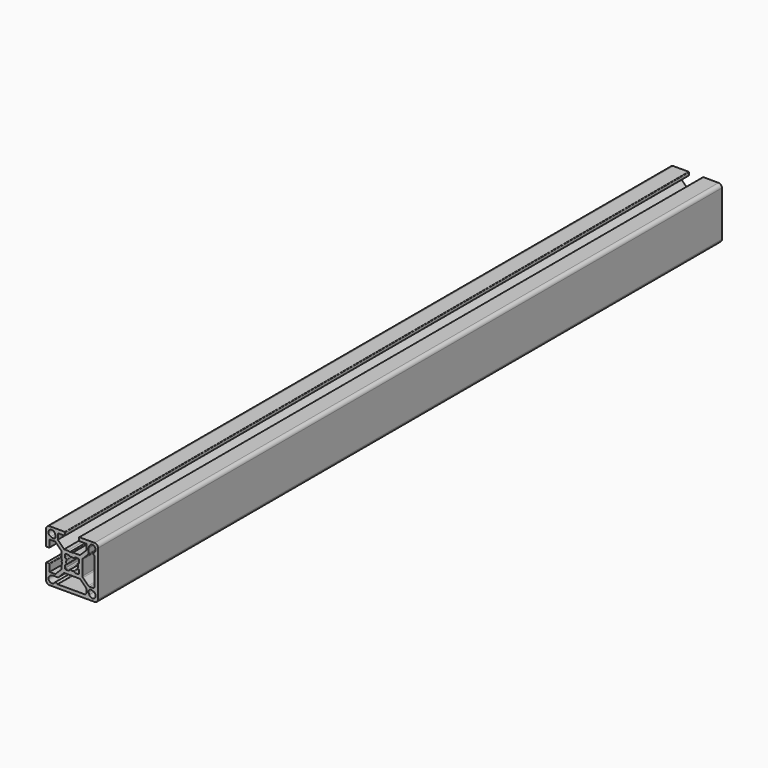
from build123d import *

# Parameters (mm, degrees)
F2_DEPTH = 225


# Not quite as in the source:
# - ends of sketch curves that miss each other by under 0.0002 mm in the source are joined


with BuildPart() as f2:
    # F1 (on Front) → F2 (new body, symmetric)
    with BuildSketch(Plane.XZ):
        with BuildLine():
            Line((-48.090856, 20.246586), (-44.140856, 20.246586))
            ThreePointArc((-44.140856, 20.246586), (-43.9287239656, 20.3344539656), (-43.840856, 20.546586))
            Line((-43.840856, 20.546586), (-43.840856, 21.946586))
            ThreePointArc((-43.840856, 21.946586), (-43.9287239656, 22.1587180344), (-44.140856, 22.246586))
            Line((-44.140856, 22.246586), (-52.840856, 22.246586))
            ThreePointArc((-52.840856, 22.246586), (-54.2550695624, 21.6607995624), (-54.840856, 20.246586))
            Line((-54.840856, 20.246586), (-54.840856, 11.546586))
            ThreePointArc((-54.840856, 11.546586), (-54.7529880344, 11.3344539656), (-54.540856, 11.246586))
            Line((-54.540856, 11.246586), (-53.140856, 11.246586))
            ThreePointArc((-53.140856, 11.246586), (-52.9287239656, 11.3344539656), (-52.840856, 11.546586))
            Line((-52.840856, 11.546586), (-52.840856, 15.496586))
            Line((-52.840856, 15.496586), (-49.50507, 15.496586))
            Line((-49.50507, 15.496586), (-45.840856, 11.832372))
            Line((-45.840856, 11.832372), (-45.840856, 7.900176))
            ThreePointArc((-45.840856, 7.900176), (-45.8238189324, 7.7707665494), (-45.7738687764, 7.6501761291))
            Line((-45.7738687764, 7.6501761291), (-45.540856, 7.246586))
            Line((-45.540856, 7.246586), (-45.773869, 6.842996))
            ThreePointArc((-45.773869, 6.842996), (-45.840856, 6.592996), (-45.7738687764, 6.3429961291))
            Line((-45.7738687764, 6.3429961291), (-45.591833, 6.0277))
            Line((-45.591833, 6.0277), (-45.840856, 4.746586))
            Line((-45.840856, 4.746586), (-45.840856, 2.6608))
            Line((-45.840856, 2.6608), (-49.50507, -1.003414))
            Line((-49.50507, -1.003414), (-52.840856, -1.003414))
            Line((-52.840856, -1.003414), (-52.840856, 2.946586))
            ThreePointArc((-52.840856, 2.946586), (-52.9287239656, 3.1587180344), (-53.140856, 3.246586))
            Line((-53.140856, 3.246586), (-54.540856, 3.246586))
            ThreePointArc((-54.540856, 3.246586), (-54.7529880344, 3.1587180344), (-54.840856, 2.946586))
            Line((-54.840856, 2.946586), (-54.840856, -5.753414))
            ThreePointArc((-54.840856, -5.753414), (-54.2550695624, -7.1676275624), (-52.840856, -7.753414))
            Line((-52.840856, -7.753414), (-26.840856, -7.753414))
            ThreePointArc((-26.840856, -7.753414), (-25.4266424376, -7.1676275624), (-24.840856, -5.753414))
            Line((-24.840856, -5.753414), (-24.840856, 20.246586))
            ThreePointArc((-24.840856, 20.246586), (-25.4266424376, 21.6607995624), (-26.840856, 22.246586))
            Line((-26.840856, 22.246586), (-35.540856, 22.246586))
            ThreePointArc((-35.540856, 22.246586), (-35.7529880344, 22.1587180344), (-35.840856, 21.946586))
            Line((-35.840856, 21.946586), (-35.840856, 20.546586))
            ThreePointArc((-35.840856, 20.546586), (-35.7529880344, 20.3344539656), (-35.540856, 20.246586))
            Line((-35.540856, 20.246586), (-31.590856, 20.246586))
            Line((-31.590856, 20.246586), (-31.590856, 16.9108))
            Line((-31.590856, 16.9108), (-35.25507, 13.246586))
            Line((-35.25507, 13.246586), (-39.187266, 13.246586))
            ThreePointArc((-39.187266, 13.246586), (-39.3166754506, 13.2295489324), (-39.4372658709, 13.1795987764))
            Line((-39.4372658709, 13.1795987764), (-39.840856, 12.946586))
            Line((-39.840856, 12.946586), (-40.244446, 13.179599))
            ThreePointArc((-40.244446, 13.179599), (-40.494446, 13.246586), (-40.7444458709, 13.1795987764))
            Line((-40.7444458709, 13.1795987764), (-41.059742, 12.997563))
            Line((-41.059742, 12.997563), (-42.340856, 13.246586))
            Line((-42.340856, 13.246586), (-44.426642, 13.246586))
            Line((-44.426642, 13.246586), (-48.090856, 16.9108))
            Line((-48.090856, 16.9108), (-48.090856, 20.246586))
        make_face()
        with BuildLine():
            ThreePointArc((-48.030175, -5.753414), (-48.180175082, -5.7132215738), (-48.2899827159, -5.6034138359))
            ThreePointArc((-48.2899827159, -5.6034138359), (-49.1151948384, -5.1042472042), (-49.9783690315, -5.5344479782))
            ThreePointArc((-49.9783690315, -5.5344479782), (-53.0449723505, -5.6142903949), (-52.1906940253, -2.6679979306))
            Line((-52.1906940253, -2.6679979306), (-50.91426, -2.203414))
            Line((-50.91426, -2.203414), (-48.290856, -2.203414))
            ThreePointArc((-48.290856, -2.203414), (-47.9081725676, -2.1272935325), (-47.5837492188, -1.9105207812))
            Line((-47.5837492188, -1.9105207812), (-44.719536, 0.953693))
            ThreePointArc((-44.719536, 0.953693), (-44.3951124324, 1.1704655325), (-44.012429, 1.246586))
            Line((-44.012429, 1.246586), (-35.669283, 1.246586))
            ThreePointArc((-35.669283, 1.246586), (-35.2865995676, 1.1704655325), (-34.9621762188, 0.9536927812))
            Line((-34.9621762188, 0.9536927812), (-31.883749, -2.124734))
            ThreePointArc((-31.883749, -2.124734), (-31.6669764675, -2.4491575676), (-31.590856, -2.831841))
            Line((-31.590856, -2.831841), (-31.590856, -4.753414))
            ThreePointArc((-31.590856, -4.753414), (-31.8837492188, -5.4605207812), (-32.590856, -5.753414))
            Line((-32.590856, -5.753414), (-48.030175, -5.753414))
        make_face(mode=Mode.SUBTRACT)
        with BuildLine():
            ThreePointArc((-30.2930043339, -4.0956641215), (-29.9673844937, -2.6268855063), (-28.4986058785, -2.3012656661))
            Line((-28.4986058785, -2.3012656661), (-27.491018, -2.667998))
            ThreePointArc((-27.491018, -2.667998), (-26.7973531157, -5.7969168843), (-29.9262720694, -5.1032520253))
            Line((-29.9262720694, -5.1032520253), (-30.2930043339, -4.0956641215))
        make_face(mode=Mode.SUBTRACT)
        with BuildLine():
            ThreePointArc((-36.5876690145, 8.2349049956), (-36.440856, 7.246586), (-36.5876690145, 6.2582670044))
            ThreePointArc((-36.5876690145, 6.2582670044), (-36.5433888407, 5.9288023569), (-36.2653470651, 5.7465855742))
            ThreePointArc((-36.2653470651, 5.7465855742), (-35.9615444769, 5.5780848975), (-35.840856, 5.25232))
            Line((-35.840856, 5.25232), (-35.840856, 3.746586))
            ThreePointArc((-35.840856, 3.746586), (-35.9873026094, 3.3930326094), (-36.340856, 3.246586))
            Line((-36.340856, 3.246586), (-37.84659, 3.246586))
            ThreePointArc((-37.84659, 3.246586), (-38.1723548975, 3.3672744769), (-38.3408555178, 3.6710770737))
            ThreePointArc((-38.3408555178, 3.6710770737), (-38.5230723569, 3.9491188407), (-38.8525409519, 3.9933978415))
            ThreePointArc((-38.8525409519, 3.9933978415), (-39.840856, 3.846586), (-40.8291749956, 3.9933990145))
            ThreePointArc((-40.8291749956, 3.9933990145), (-41.1586396431, 3.9491188407), (-41.3408564258, 3.6710770651))
            ThreePointArc((-41.3408564258, 3.6710770651), (-41.5093571025, 3.3672744769), (-41.835122, 3.246586))
            Line((-41.835122, 3.246586), (-43.340856, 3.246586))
            ThreePointArc((-43.340856, 3.246586), (-43.6944093906, 3.3930326094), (-43.840856, 3.746586))
            Line((-43.840856, 3.746586), (-43.840856, 5.25232))
            ThreePointArc((-43.840856, 5.25232), (-43.7201675231, 5.5780848975), (-43.4163649263, 5.7465855178))
            ThreePointArc((-43.4163649263, 5.7465855178), (-43.1383231593, 5.9288023569), (-43.0940441585, 6.2582709519))
            ThreePointArc((-43.0940441585, 6.2582709519), (-43.240856, 7.246586), (-43.0940429855, 8.2349049956))
            ThreePointArc((-43.0940429855, 8.2349049956), (-43.1383231593, 8.5643696431), (-43.4163649349, 8.7465864258))
            ThreePointArc((-43.4163649349, 8.7465864258), (-43.7201675231, 8.9150871025), (-43.840856, 9.240852))
            Line((-43.840856, 9.240852), (-43.840856, 10.746586))
            ThreePointArc((-43.840856, 10.746586), (-43.6944093906, 11.1001393906), (-43.340856, 11.246586))
            Line((-43.340856, 11.246586), (-41.835122, 11.246586))
            ThreePointArc((-41.835122, 11.246586), (-41.5093571025, 11.1258975231), (-41.3408564822, 10.8220949263))
            ThreePointArc((-41.3408564822, 10.8220949263), (-41.1586396431, 10.5440531593), (-40.8291710481, 10.4997741585))
            ThreePointArc((-40.8291710481, 10.4997741585), (-39.840856, 10.646586), (-38.8525370044, 10.4997729855))
            ThreePointArc((-38.8525370044, 10.4997729855), (-38.5230723569, 10.5440531593), (-38.3408555742, 10.8220949349))
            ThreePointArc((-38.3408555742, 10.8220949349), (-38.1723548975, 11.1258975231), (-37.84659, 11.246586))
            Line((-37.84659, 11.246586), (-36.340856, 11.246586))
            ThreePointArc((-36.340856, 11.246586), (-35.9873026094, 11.1001393906), (-35.840856, 10.746586))
            Line((-35.840856, 10.746586), (-35.840856, 9.240852))
            ThreePointArc((-35.840856, 9.240852), (-35.9615444769, 8.9150871025), (-36.2653470737, 8.7465864822))
            ThreePointArc((-36.2653470737, 8.7465864822), (-36.5433888407, 8.5643696431), (-36.5876690145, 8.2349049956))
        make_face(mode=Mode.SUBTRACT)
        with BuildLine():
            ThreePointArc((-49.3887076661, 18.5888361215), (-49.7143275063, 17.1200575063), (-51.1831061215, 16.7944376661))
            Line((-51.1831061215, 16.7944376661), (-52.190694, 17.16117))
            ThreePointArc((-52.190694, 17.16117), (-52.8843588843, 20.2900888843), (-49.7554399306, 19.5964240253))
            Line((-49.7554399306, 19.5964240253), (-49.3887076661, 18.5888361215))
        make_face(mode=Mode.SUBTRACT)
        with BuildLine():
            ThreePointArc((-33.5479627812, 2.3679062188), (-33.7647355325, 2.6923295676), (-33.840856, 3.075013))
            Line((-33.840856, 3.075013), (-33.840856, 11.418159))
            ThreePointArc((-33.840856, 11.418159), (-33.7647355325, 11.8008424324), (-33.5479627812, 12.1252657812))
            Line((-33.5479627812, 12.1252657812), (-30.683749, 14.989479))
            ThreePointArc((-30.683749, 14.989479), (-30.4669764675, 15.3139025676), (-30.390856, 15.696586))
            Line((-30.390856, 15.696586), (-30.390856, 18.31999))
            Line((-30.390856, 18.31999), (-29.926272, 19.596424))
            ThreePointArc((-29.926272, 19.596424), (-26.9799796051, 20.4507023505), (-27.0598220201, 17.3840990291))
            ThreePointArc((-27.0598220201, 17.3840990291), (-27.4900227958, 16.5209248384), (-26.9908561748, 15.6957126972))
            ThreePointArc((-26.9908561748, 15.6957126972), (-26.8810484262, 15.585905082), (-26.840856, 15.435905))
            Line((-26.840856, 15.435905), (-26.840856, -0.003414))
            ThreePointArc((-26.840856, -0.003414), (-27.1337492188, -0.7105207812), (-27.840856, -1.003414))
            Line((-27.840856, -1.003414), (-29.762429, -1.003414))
            ThreePointArc((-29.762429, -1.003414), (-30.1451124324, -0.9272935325), (-30.4695357812, -0.7105207812))
            Line((-30.4695357812, -0.7105207812), (-33.5479627812, 2.3679062188))
        make_face(mode=Mode.SUBTRACT)
    extrude(amount=F2_DEPTH, both=True)


solid = f2.part
